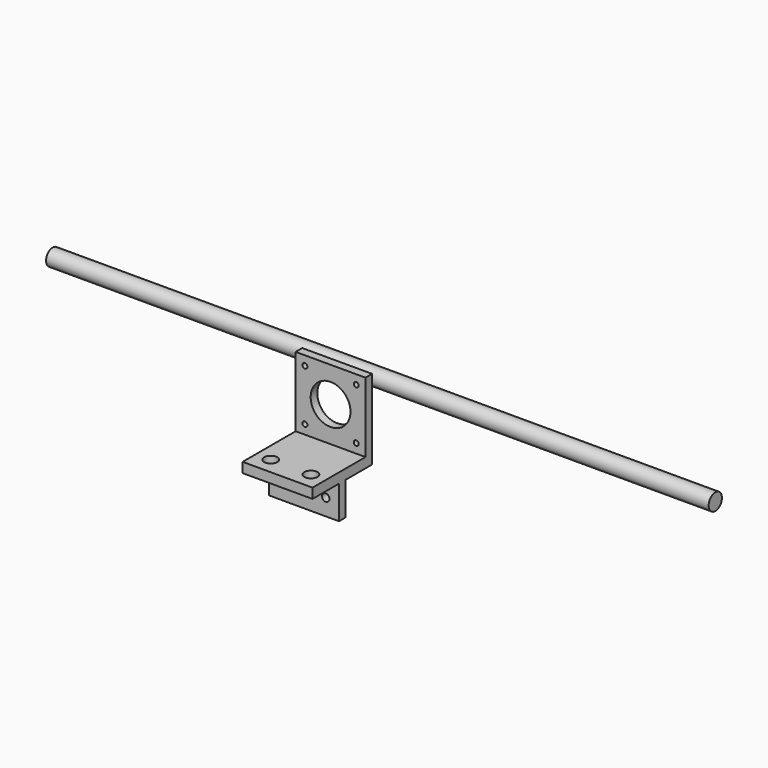
from build123d import *

# Parameters (mm, degrees)
F0_W      = 42.18
F0_H      = 6
F0_H_2    = 42.18
F0_R      = 1.5
F0_R_2    = 12.01
F1_DEPTH  = 5
F2_W      = 42.18
F2_H      = 6
F3_DEPTH  = 40
F4_R      = 2.25
F5_DEPTH  = 6
F6_R      = 4
F6_R_2    = 2.25
F7_DEPTH  = 5
F8_W      = 42.18
F8_H      = 5
F9_DEPTH  = 20
F10_R     = 2.25
F11_DEPTH = 5
F12_R     = 5
F13_DEPTH = 200


# Not quite as in the source:
# - a feature names something its author has since deleted; it is built from what else it names


with BuildPart() as f1:
    # F0 (on Front) → F1 (new body)
    with BuildSketch(Plane.XZ):
        with Locations((0, -21.09)):
            Rectangle(F0_W, F0_H)
        with Locations((0, 3)):
            Rectangle(F0_W, F0_H_2)
        with Locations((-15.5, -12.5)):
            Circle(F0_R, mode=Mode.SUBTRACT)
        with Locations((15.5, -12.5)):
            Circle(F0_R, mode=Mode.SUBTRACT)
        with Locations((-15.5, 18.5)):
            Circle(F0_R, mode=Mode.SUBTRACT)
        with Locations((0, 3)):
            Circle(F0_R_2, mode=Mode.SUBTRACT)
        with Locations((15.5, 18.5)):
            Circle(F0_R, mode=Mode.SUBTRACT)
    extrude(amount=F1_DEPTH)

    # F2 (on face) → F3 (join)
    with BuildSketch(Plane.XZ.offset(5)):
        with Locations((0, -21.09)):
            Rectangle(F2_W, F2_H)
    extrude(amount=F3_DEPTH)

    # F4 (on face) → F5 (cut, through all)
    with BuildSketch(Plane.XY.offset(-18.09)):
        with Locations((-12.115384452, -35)):
            Circle(F4_R)
        with Locations((12.115384452, -35)):
            Circle(F4_R)
    extrude(amount=-F5_DEPTH, mode=Mode.SUBTRACT)

    # F6 (on face) → F7 (cut)
    with BuildSketch(Plane.XY.offset(-18.09)):
        with Locations((-12.115384452, -35)):
            Circle(F6_R)
        with Locations((-12.115384452, -35)):
            Circle(F6_R_2, mode=Mode.SUBTRACT)
        with Locations((12.115384452, -35)):
            Circle(F6_R)
        with Locations((12.115384452, -35)):
            Circle(F6_R_2, mode=Mode.SUBTRACT)
    extrude(amount=-F7_DEPTH, mode=Mode.SUBTRACT)

    # F8 (on face) → F9 (join)
    with BuildSketch(Plane(origin=(0, 0, -24.09), x_dir=(1, 0, 0), z_dir=(0, 0, -1))):
        with Locations((0, 22.5)):
            Rectangle(F8_W, F8_H)
    extrude(amount=F9_DEPTH)

    # F10 (on face) → F11 (cut, through all)
    with BuildSketch(Plane(origin=(0, -20, 0), x_dir=(-1, 0, 0), z_dir=(0, 1, 0))):
        with Locations((13.09, -34.09)):
            Circle(F10_R)
        with Locations((-13.09, -34.09)):
            Circle(F10_R)
    extrude(amount=-F11_DEPTH, mode=Mode.SUBTRACT)


with BuildPart() as f13:
    # F12 (on Right) → F13 (new body, symmetric)
    with BuildSketch(Plane.YZ):
        with Locations((35.3150554001, 0)):
            Circle(F12_R)
    extrude(amount=F13_DEPTH, both=True)


solid = Compound([f1.part, f13.part])
